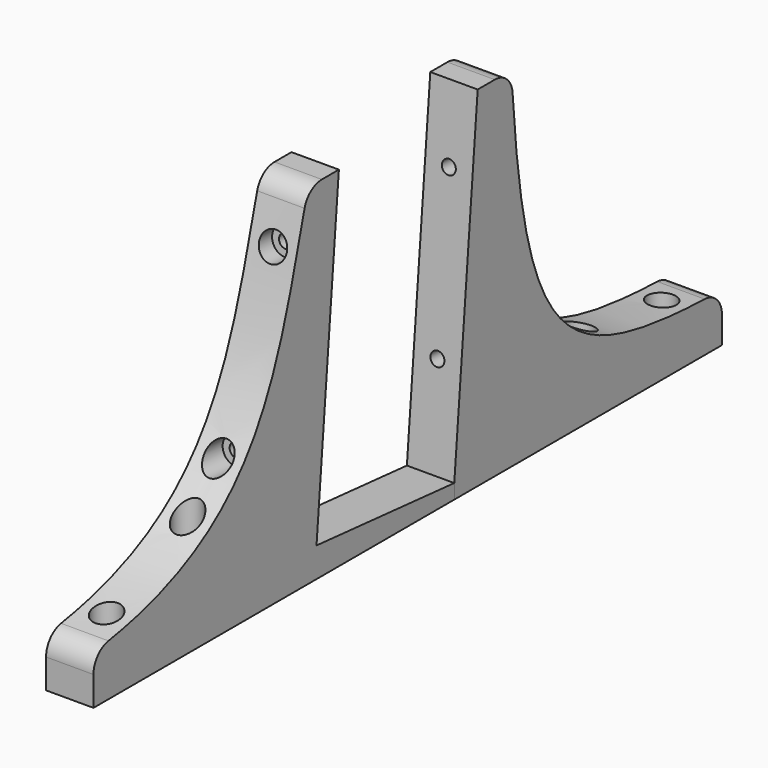
from build123d import *

# Parameters (mm, degrees)
F1_DEPTH          = 17
F2_DEPTH          = 17
F3_R              = 8
F3_2_R            = 8
F6_D              = 5
F6_START          = 19.6170088
F6_START_2        = 36.716643
F6_CBORE_D        = 10
F6_CBORE_DEPTH    = 5
F9_D              = 5
F9_START          = 26.9055071
F9_START_2        = 49.0819507
F9_CBORE_D        = 10
F9_CBORE_DEPTH    = 5
F12_D             = 5
F12_START         = 40.6627689
F12_START_2       = 50.2635382
F12_START_3       = 53.9077982
F12_START_4       = 55.3815003
F12_CBORE_D       = 10
F12_CBORE_DEPTH   = 5
F12_2_D           = 5
F12_2_START       = 40.6627689
F12_2_START_2     = 50.2635382
F12_2_START_3     = 53.9077982
F12_2_START_4     = 55.3815003
F12_2_CBORE_D     = 10
F12_2_CBORE_DEPTH = 5


with BuildPart() as f1:
    # F0 (on Right) → F1 (new body)
    with BuildSketch(Plane.YZ):
        with BuildLine():
            Line((61.7640712817, -5.4036560504), (0, 0))
            Line((0, 0), (10.0258809771, 114.5963439496))
            Line((10.0258809771, 114.5963439496), (-3.7634782237, 114.5963439496))
            add(Edge.make_bspline(
                [(-3.7634782237, 114.5963439496), (-18.0635154247, 61.5457296371), (-24.2072818387, 16.3963653548), (-100, 6.8306473353)],
                knots=[0, 0, 0, 0, 144.4815333888, 144.4815333888, 144.4815333888, 144.4815333888], degree=3))
            Line((-100, 6.8306473353), (-100, -5.4036560504))
            Line((-100, -5.4036560504), (-100, -10.6361983344))
            Line((-100, -10.6361983344), (61.7640712817, -10.6361983344))
            Line((61.7640712817, -10.6361983344), (61.7640712817, -5.4036560504))
        make_face()
    extrude(amount=F1_DEPTH)

    # F3
    f3_edges = [f1.edges().sort_by_distance(p)[0] for p in [
        (8.5, -100, 6.830647),
        (8.5, -3.763478, 114.596344),
    ]]
    fillet(f3_edges, radius=F3_R)

    # F6 (through all)
    # its depths count from where the whole tool has entered the part; down to there all is cleared
    with Locations(Plane(origin=(0, -52.7983189989, 4.6192543656), x_dir=(-1, 0, 0), z_dir=(0, -0.9961946981, 0.0871557427))):
        with Locations((-8.5, -94.0341213839, -F6_START_2), (-8.5, -35.3030460076, -F6_START)):
            CounterBoreHole(F6_D / 2, F6_CBORE_D / 2, F6_CBORE_DEPTH)

    # F12 (through all)
    # its depths count from where the whole tool has entered the part; down to there all is cleared
    with Locations(Plane.XY.offset(62.5638016656)):
        with Locations((8.5, 128.7754178047, -F12_START_2), (8.5, 165.3779894114, -F12_START_4), (8.5, -83.4794938564, -F12_START_3), (8.5, -47.1699088812, -F12_START)):
            CounterBoreHole(F12_D / 2, F12_CBORE_D / 2, F12_CBORE_DEPTH)


with BuildPart() as f2:
    # F0 (on Right) → F2 (new body)
    with BuildSketch(Plane.YZ):
        with BuildLine():
            Line((72.2627109048, 114.5963439496), (61.7640712817, -5.4036560504))
            Line((61.7640712817, -5.4036560504), (61.7640712817, -10.6361983344))
            Line((61.7640712817, -10.6361983344), (181.7640712817, -10.6361983344))
            Line((181.7640712817, -10.6361983344), (181.7640712817, -5.4036560504))
            Line((181.7640712817, -5.4036560504), (181.7640712817, 6.8306473353))
            add(Edge.make_bspline(
                [(87.4243378639, 114.5963439496), (93.0270627141, 21.6286424547), (110.8914837241, 8.1839486957), (181.7640712817, 6.8306473353)],
                knots=[0, 0, 0, 0, 143.2251048808, 143.2251048808, 143.2251048808, 143.2251048808], degree=3))
            Line((87.4243378639, 114.5963439496), (72.2627109048, 114.5963439496))
        make_face()
    extrude(amount=F2_DEPTH)

    # F3#2
    f3_2_edges = [f2.edges().sort_by_distance(p)[0] for p in [
        (8.5, 87.424338, 114.596344),
        (8.5, 181.764071, 6.830647),
    ]]
    fillet(f3_2_edges, radius=F3_2_R)

    # F9 (through all)
    # its depths count from where the whole tool has entered the part; down to there all is cleared
    with Locations(Plane(origin=(0, 129.5053107519, -11.3302465572), x_dir=(1, 0, 0), z_dir=(0, 0.9961946981, -0.0871557427))):
        with Locations((8.5, -94.0341213839, -F9_START_2), (8.5, -35.3030460076, -F9_START)):
            CounterBoreHole(F9_D / 2, F9_CBORE_D / 2, F9_CBORE_DEPTH)

    # F12#2 (through all)
    # its depths count from where the whole tool has entered the part; down to there all is cleared
    with Locations(Plane.XY.offset(62.5638016656)):
        with Locations((8.5, 128.7754178047, -F12_2_START_2), (8.5, 165.3779894114, -F12_2_START_4), (8.5, -83.4794938564, -F12_2_START_3), (8.5, -47.1699088812, -F12_2_START)):
            CounterBoreHole(F12_2_D / 2, F12_2_CBORE_D / 2, F12_2_CBORE_DEPTH)


solid = Compound([f1.part, f2.part])
